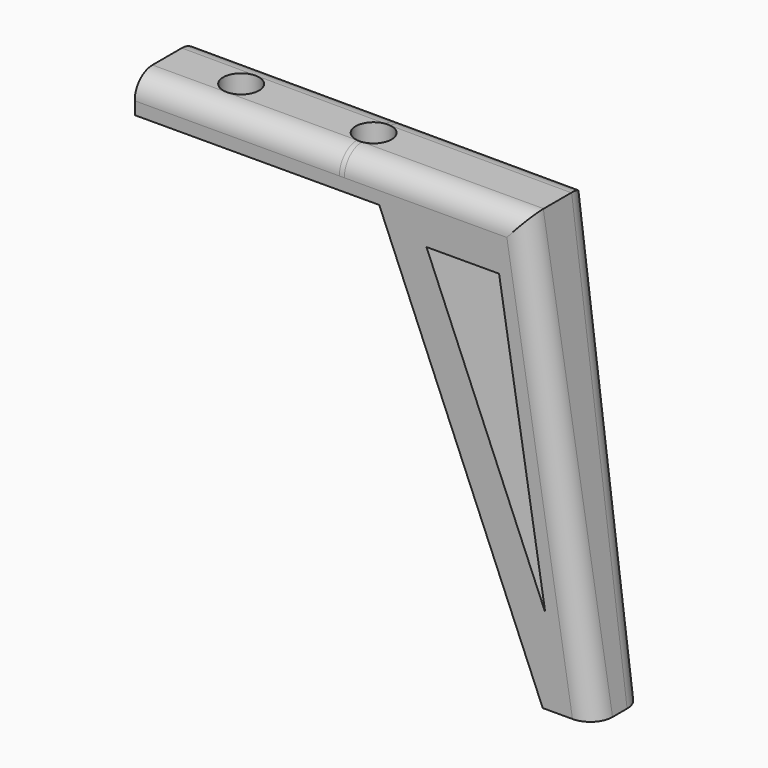
from build123d import *

# Parameters (mm, degrees)
F1_DEPTH      = 11.5
F1_DEPTH_BACK = 7.25
F4_DEPTH      = 57.75
F5_R          = 2.032
F6_DEPTH      = 25
F7_R          = 2.5


# Not quite as in the source:
# - a feature names something its author has since deleted; it is built from what else it names


with BuildPart() as f1:
    # F0 (on Front) → F1 (new body, two sides)
    with BuildSketch(Plane.XZ) as f1_sk:
        Polygon((-26.8014297359, 2.0000000475), (-26.8014297359, -2.0000000475), (0.7941166829, -2.0000000475), (18.5593261492, -46.7420644607), (24.4487996128, -46.7420644607), (17.3888709152, 2.0000000475), align=None)
        Polygon((18.9966002603, -37.0041966029), (6.0891124744, -4.4964093445), (14.2880869367, -4.4964093445), align=None, mode=Mode.SUBTRACT)
    extrude(amount=F1_DEPTH)
    extrude(f1_sk.sketch, amount=-F1_DEPTH_BACK)

    # F3 (on offset) → F4 (cut)
    with BuildSketch(Plane(origin=(18.7998007554, 0, 2.7230125396), x_dir=(0, 1, 0), z_dir=(0.9896725236, 0, 0.1433467688))):
        Polygon((-18.5980091819, 10.2755831857), (-17.1822748397, -51.6943840463), (-3.4891957167, -51.8214939905), (-4.7216577223, 10.5497811385), align=None)
        Polygon((3.4891957167, -51.8214939905), (17.1822748397, -51.6943840463), (18.5980091819, 10.2755831857), (4.7216577223, 10.5497811385), align=None)
    extrude(amount=-F4_DEPTH, mode=Mode.SUBTRACT)

    # F5 (on face) → F6 (cut)
    with BuildSketch(Plane.XY.offset(2.0000000475)):
        with Locations((-3.4189070485, 0)):
            Circle(F5_R)
        with Locations((-18.4189070485, 0)):
            Circle(F5_R)
    extrude(amount=-F6_DEPTH, mode=Mode.SUBTRACT)

    # F7
    f7_edges = [f1.edges().sort_by_distance(p)[0] for p in [
        (-4.706279, -4.565636, 2),
        (-4.706279, 4.565636, 2),
        (20.918835, 4.016451, -22.371032),
        (20.918835, -4.016451, -22.371032),
    ]]
    fillet(f7_edges, radius=F7_R)


solid = f1.part
